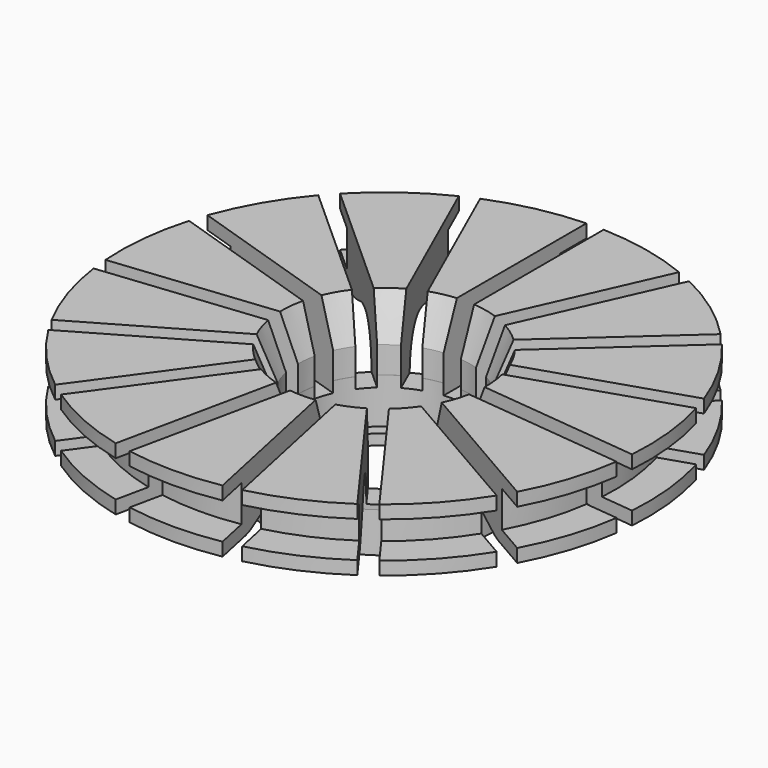
from build123d import *

# Parameters (mm, degrees)
F3_W            = 3.3156562131
F3_H            = 17.2335729003
F4_DEPTH        = 76.2
F4_COPIES_COUNT = 15


# Not quite as in the source:
# - a pattern or mirror of a feature is missing from the dataset's text; its kind, count and spacing are read off the source's solid


with BuildPart() as f1:
    # F0 (on Front) → F1 (revolve)
    with BuildSketch(Plane.XZ):
        with BuildLine():
            Line((43.2148316451, 87.9881810245), (50.8000223151, 87.9881810245))
            Line((50.8000223151, 87.9881810245), (50.8000223151, 90.5281810245))
            Line((50.8000223151, 90.5281810245), (44.45, 90.5281810245))
            Line((44.45, 90.5281810245), (44.45, 97.5131810245))
            Line((44.45, 97.5131810245), (49.53, 97.5131810245))
            Line((49.53, 97.5131810245), (50.8000223151, 97.5131810245))
            Line((50.8000223151, 97.5131810245), (50.8000223151, 100.0531810245))
            Line((50.8000223151, 100.0531810245), (49.53, 100.0531810245))
            Line((49.53, 100.0531810245), (19.685, 100.0531810245))
            Line((19.685, 100.0531810245), (16.51, 92.0810773969))
            Line((16.51, 92.0810773969), (16.51, 86.9589045931))
            ThreePointArc((16.51, 86.9589045931), (16.5100223151, 86.9452022966), (16.51, 86.9315))
            Line((16.51, 86.9315), (16.51, 78.2340656991))
            Line((16.51, 78.2340656991), (15.882236624, 78.2340656991))
            Line((15.882236624, 78.2340656991), (14.2875223151, 78.2340656991))
            Line((14.2875223151, 78.2340656991), (14.2875223151, 76.2020656991))
            Line((14.2875223151, 76.2020656991), (21.59, 76.2020656991))
            Line((21.59, 76.2020656991), (21.59, 83.9149579406))
            add(Edge.make_bspline(
                [(43.2148316451, 87.9881810245), (41.901504392, 87.9881810245), (40.1127141517, 88.6171544634), (38.6895401079, 88.9345218172), (36.4095956769, 89.6466679596), (32.8491492058, 91.0777258122), (30.4619169323, 92.2515961562), (26.776241714, 92.7515877358), (23.7400971585, 91.4449247158), (21.746825787, 88.4740279898), (21.59, 83.9149579406)],
                knots=[0, 0, 0, 0, 0.1239588066, 0.2051945126, 0.3108268963, 0.4461545989, 0.5613140183, 0.6904091481, 0.8050620964, 1, 1, 1, 1], degree=3))
        make_face()
    revolve(axis=Axis((2.23151e-05, 0, 91.5753121757), (0, 0, 1)))

    # F3 (on offset) → F4 (cut)
    with BuildSketch(Plane.XZ.offset(-6.35)):
        with Locations((0, 93.4582985938)):
            Rectangle(F3_W, F3_H)
    f4 = extrude(amount=-F4_DEPTH, mode=Mode.SUBTRACT)

    # F4_copies: F4 ×15 about axis
    f4_copies_axis = Axis((0, 0, 0), (0, 0, 1))
    for i in range(1, F4_COPIES_COUNT):
        add(f4.rotate(f4_copies_axis, i * 360 / F4_COPIES_COUNT), mode=Mode.SUBTRACT)


solid = f1.part
